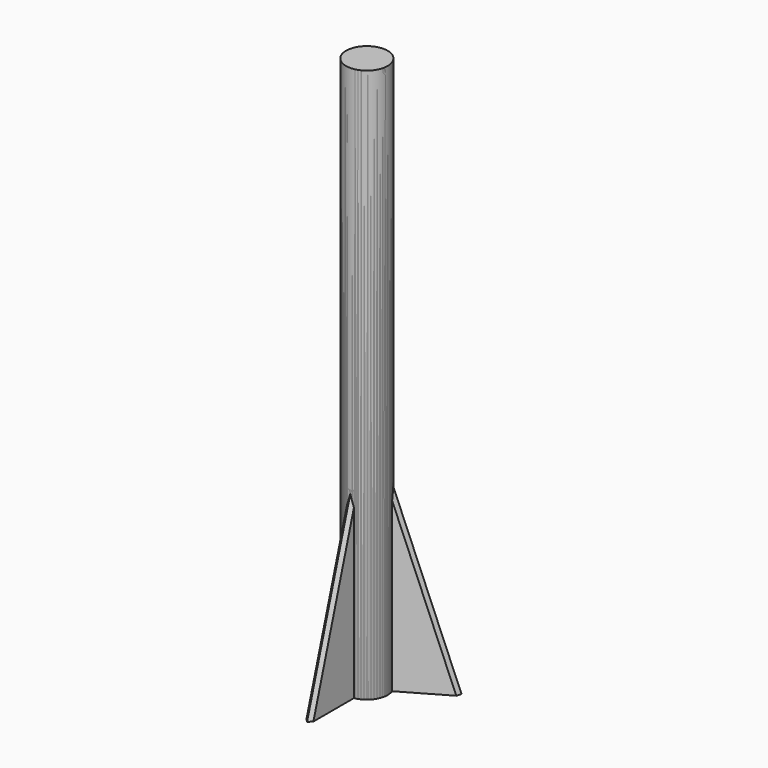
from build123d import *

# Parameters (mm, degrees)
F0_R         = 9.525
F1_DEPTH     = 254
F2_W         = 3.213812945
F2_H         = 83.5626572371
F3_DEPTH     = 1.5875
F4_T4_DEPTH  = 97.7399238564
F4_S5_R      = 9.525
F4_T6_DEPTH  = 51
F4_T10_DEPTH = 97.7399238564
F4_S11_R     = 9.525
F4_T12_DEPTH = 51
F5_COUNT     = 3


# Not quite as in the source:
# - a fillet or chamfer that OpenCascade refuses, or shapes differently, is made with other operations: its cross-section is extruded or revolved along the edge and cut away or added


with BuildPart() as f1:
    # F0 (on Top) → F1 (new body)
    with BuildSketch(Plane.XY):
        Circle(F0_R)
    extrude(amount=F1_DEPTH)

    # F2 (on Right) → F3 (join, symmetric)
    with BuildSketch(Plane.YZ):
        Polygon((-34.7555913031, 0), (-9.525, 0), (-9.525, 83.5626572371), align=None)
        with Locations((-7.9180935275, 41.7813286185)):
            Rectangle(F2_W, F2_H)
    extrude(amount=F3_DEPTH, both=True)

    # F4: chamfer of 2.032 on 2 edges, made by hand


with BuildPart() as f4_tool2:
    # F4_s3 → F4_t4 (new body)
    with BuildSketch(Plane(origin=(0, 23.8372726248, 78.9480443752), x_dir=(1, 0, 0), z_dir=(0, -0.2890479409, -0.9573146232))):
        Polygon((1.5875, 31.240035794), (-0.4445, 33.272035794), (1.5875, 33.272035794), align=None)
    extrude(amount=F4_T4_DEPTH)

    # F4_s5 → F4_t6 (cut, symmetric)
    with BuildSketch(Plane.XY.offset(41.5)):
        Circle(F4_S5_R)
    extrude(amount=F4_T6_DEPTH, both=True, mode=Mode.SUBTRACT)


with BuildPart() as f1_1:
    add(f1.part)

    # F4_t1: cut F4_tool2
    add(f4_tool2.part, mode=Mode.SUBTRACT)


with BuildPart() as f4_tool8:
    # F4_s9 → F4_t10 (new body)
    with BuildSketch(Plane(origin=(0, 23.8372726248, 78.9480443752), x_dir=(1, 0, 0), z_dir=(0, -0.2890479409, -0.9573146232))):
        Polygon((-1.5875, 31.240035794), (0.4445, 33.272035794), (-1.5875, 33.272035794), align=None)
    extrude(amount=F4_T10_DEPTH)

    # F4_s11 → F4_t12 (cut, symmetric)
    with BuildSketch(Plane.XY.offset(41.5)):
        Circle(F4_S11_R)
    extrude(amount=F4_T12_DEPTH, both=True, mode=Mode.SUBTRACT)


with BuildPart() as f1_2:
    add(f1_1.part)

    # F4_t7: cut F4_tool8
    add(f4_tool8.part, mode=Mode.SUBTRACT)


with BuildPart() as f5_1:
    # F5: instance of F1
    add(f1_2.part.rotate(Axis((0, 0, 0), (0, 0, -1)), 1 * 360 / F5_COUNT))


with BuildPart() as f5_2:
    # F5: instance of F1
    add(f1_2.part.rotate(Axis((0, 0, 0), (0, 0, -1)), 2 * 360 / F5_COUNT))


solid = Compound([f1_2.part, f5_1.part, f5_2.part])
